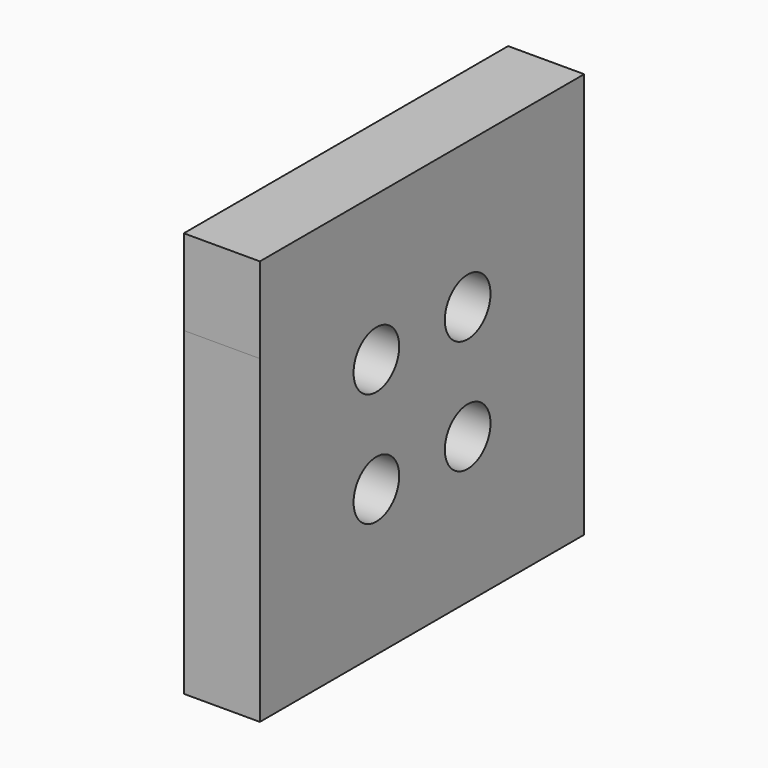
from build123d import *

# Parameters (mm, degrees)
F0_R     = 3.75
F0_W     = 11.25
F0_H     = 30.8000000767
F0_W_2   = 11.2448162399
F0_H_2   = 30.8000003636
F1_DEPTH = 10


# Not quite as in the source:
# - ends of sketch curves that miss each other by under 0.0002 mm in the source are joined


with BuildPart() as f1:
    # F0 (on Right) → F1 (new body)
    with BuildSketch(Plane.YZ):
        Polygon((11.25, 26.6500003636), (-4.1499999352, 26.6500003636), (-4.1499999352, -4.15), (11.25, -4.15), (26.65, -4.15), (26.65, 26.65), align=None)
        with Locations((3.75, 3.75)):
            Circle(F0_R, mode=Mode.SUBTRACT)
        with Locations((18.75, 3.75)):
            Circle(F0_R, mode=Mode.SUBTRACT)
        with Locations((3.75, 18.75)):
            Circle(F0_R, mode=Mode.SUBTRACT)
        with Locations((18.75, 18.75)):
            Circle(F0_R, mode=Mode.SUBTRACT)
        with Locations((32.275, 11.2500000384)):
            Rectangle(F0_W, F0_H)
        Polygon((11.25, -4.15), (-4.1499999352, -4.15), (-15.3948161751, -4.15), (-15.3948161751, -15.4), (-4.1499999352, -15.4), (26.65, -15.4), (37.9, -15.4), (37.9, -4.15), (26.65, -4.15), align=None)
        Polygon((-15.3948161751, 26.6500003636), (-4.1499999352, 26.6500002869), (11.25, 26.6500003636), (26.65, 26.65), (37.9, 26.65), (37.9000000767, 37.9), (-15.3948160984, 37.9000003636), align=None)
        with Locations((-9.7724080551, 11.2500001818)):
            Rectangle(F0_W_2, F0_H_2)
    extrude(amount=F1_DEPTH)


solid = f1.part
